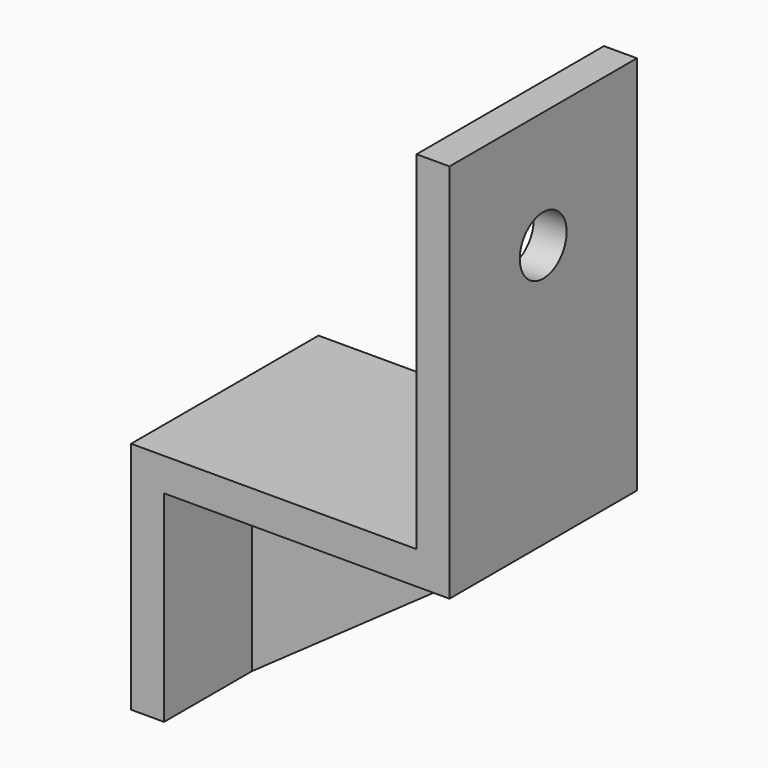
from build123d import *

# Parameters (mm, degrees)
F1_DEPTH  = 101.6
F3_D      = 25.4
F4_W      = 101.6
F4_H      = 87.3125
F5_DEPTH  = 123.825
F7_DEPTH  = 101.601
F8_W      = 151.5127165662
F8_H      = 47.625
F9_DEPTH  = 214.5206515044
F10_DEPTH = 214.5206515044


with BuildPart() as f1:
    # F0 (on Front) → F1 (new body)
    with BuildSketch(Plane.XZ):
        Polygon((-37.8673051461, 7.5604184782), (-37.8673051461, -94.0395815218), (-23.5798051461, -94.0395815218), (-23.5798051461, -6.7270815218), (100.2451948539, -6.7270815218), (100.2451948539, 158.3729184782), (85.9576948539, 158.3729184782), (85.9576948539, 7.5604184782), align=None)
    extrude(amount=F1_DEPTH)

    # F3 (through all)
    with Locations(Plane.YZ.offset(100.2451948539)):
        with Locations((-50.8, 107.5729184782)):
            Hole(F3_D / 2)


with BuildPart() as f5:
    # F4 (on face) → F5 (new body, through all)
    with BuildSketch(Plane.YZ.offset(-23.5798051461)):
        with Locations((-50.8, -50.3833315218)):
            Rectangle(F4_W, F4_H)
    extrude(amount=F5_DEPTH)

    # F6 (on face) → F7 (cut, through all)
    with BuildSketch(Plane.XZ.offset(101.6)):
        Polygon((100.2451948539, -6.7270815218), (-23.5798051461, -94.0395815218), (100.2451948539, -94.0395815218), align=None)
    extrude(amount=-F7_DEPTH, mode=Mode.SUBTRACT)

    # F8 (on face) → F9 (cut, through all)
    with BuildSketch(Plane(origin=(36.4585458515, 0, -51.704846844), x_dir=(0.8172581339, 0, 0.5762717611), z_dir=(0.5762717611, 0, -0.8172581339))):
        with Locations((2.2932154783, 77.7875)):
            Rectangle(F8_W, F8_H)
    extrude(amount=-F9_DEPTH, mode=Mode.SUBTRACT)

    # F8 (on face) → F10 (cut, through all)
    with BuildSketch(Plane(origin=(36.4585458515, 0, -51.704846844), x_dir=(0.8172581339, 0, 0.5762717611), z_dir=(0.5762717611, 0, -0.8172581339))):
        with Locations((2.2932154783, 23.8125)):
            Rectangle(F8_W, F8_H)
    extrude(amount=-F10_DEPTH, mode=Mode.SUBTRACT)


solid = Compound([f1.part, f5.part])
